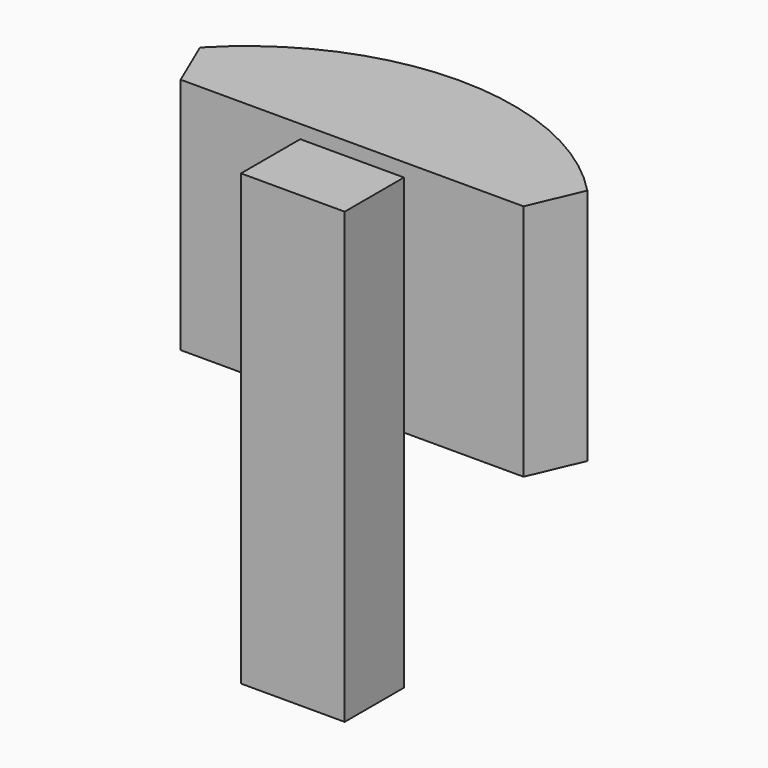
from build123d import *

# Parameters (mm, degrees)
F2_DEPTH    = 11.43
F0_W        = 4.9775806256
F0_H        = 21.5646
F3_DEPTH    = 3.556
F4_T1_DEPTH = 27.2262824301


# Not quite as in the source:
# - a fillet or chamfer that OpenCascade refuses, or shapes differently, is made with other operations: its cross-section is extruded or revolved along the edge and cut away or added


with BuildPart() as f2:
    # F1 (on Top) → F2 (new body)
    with BuildSketch(Plane.XY):
        with BuildLine():
            ThreePointArc((11.1534688622, 0), (0, 6.4792498177), (-11.1534688622, 0))
            Line((-11.1534688622, 0), (11.1534688622, 0))
        make_face()
    extrude(amount=F2_DEPTH)

    # F0 (on Front) → F3 (join)
    with BuildSketch(Plane.XZ):
        Rectangle(F0_W, F0_H)
    extrude(amount=F3_DEPTH)

    # F4: chamfer of 2.54 on 2 edges, made by hand

    # F4_s2 → F4_t1 (cut)
    with BuildSketch(Plane.XY.offset(-7.898141215)):
        with BuildLine():
            Line((-8.190415898, -0.0933816317), (-9.3391430842, 2.5863339915))
            Line((-9.3391430842, 2.5863339915), (-9.3759354233, 2.6213620343))
            ThreePointArc((-9.3759354233, 2.6213620343), (-10.327366328, 1.3537144774), (-11.1975980412, 0.0251645696))
            Line((-11.1975980412, 0.0251645696), (-11.1534688622, -0.0508))
            ThreePointArc((-11.1534688622, -0.0508), (-9.6719423801, -0.0508), (-8.190415898, -0.1441816317))
            Line((-8.190415898, -0.1441816317), (-8.190415898, -0.0933816317))
        make_face()
        with BuildLine():
            Line((8.190415898, -0.0933816317), (9.3391430842, 2.5863339915))
            Line((9.3391430842, 2.5863339915), (9.3759354233, 2.6213620343))
            ThreePointArc((9.3759354233, 2.6213620343), (10.327366328, 1.3537144774), (11.1975980412, 0.0251645696))
            Line((11.1975980412, 0.0251645696), (11.1534688622, -0.0508))
            ThreePointArc((11.1534688622, -0.0508), (9.6719423801, -0.0508), (8.190415898, -0.1441816317))
            Line((8.190415898, -0.1441816317), (8.190415898, -0.0933816317))
        make_face()
    extrude(amount=F4_T1_DEPTH, mode=Mode.SUBTRACT)


solid = f2.part
